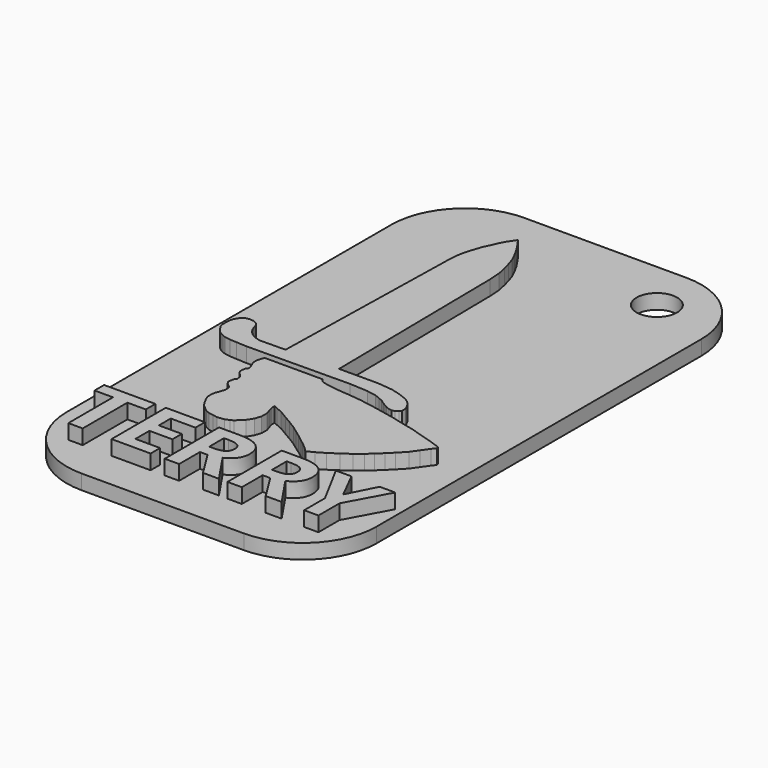
from build123d import *

# Parameters (mm, degrees)
F1_DEPTH     = 2
F3_DEPTH     = 2
F4_TEXT_SIZE = 12.8735775231
F5_DEPTH     = 2
F6_R         = 2.75
F7_DEPTH     = 25


# Not quite as in the source:
# - Text() gives the source's letters only with a copy of the font that has no kerning and outlines rounded to 1/6400 em; it was checked with that copy


with BuildPart() as f1:
    # F0 (on Top) → F1 (new body)
    with BuildSketch(Plane.XY):
        with BuildLine():
            Line((-32, 0), (-10, 0))
            ThreePointArc((-10, 0), (-2.9289321881, 2.9289321881), (0, 10))
            Line((0, 10), (0, 65))
            ThreePointArc((0, 65), (-2.9289321881, 72.0710678119), (-10, 75))
            Line((-10, 75), (-32, 75))
            ThreePointArc((-32, 75), (-39.0710678119, 72.0710678119), (-42, 65))
            Line((-42, 65), (-42, 10))
            ThreePointArc((-42, 10), (-39.0710678119, 2.9289321881), (-32, 0))
        make_face()
    extrude(amount=F1_DEPTH)

    # F2 (on face) → F3 (join)
    with BuildSketch(Plane.XY.offset(2)):
        Polygon((-24.9658841423, 16.3784821588), (-24.6103350073, 16.5639445186), (-23.6864611506, 17.4445118755), (-23.1667812914, 18.2529017329), (-22.8780712932, 19.11903359), (-22.8780712932, 20.0573448092), (-23.1523457915, 20.8657346666), (-23.2822652906, 21.4142855257), (-23.2822652906, 21.8184795231), (-22.8058937937, 21.6019470245), (-21.8964535743, 21.212188527), (-20.8426602185, 20.5770246685), (-19.7022520006, 19.9129898101), (-18.7206342816, 19.3066969514), (-17.8978089243, 18.7004040927), (-17.0172415674, 18.079675734), (-16.2377227098, 17.4589473754), (-15.6025588512, 16.9825740159), (-14.7941680625, 16.3041036576), (-14.2744891346, 15.7555527985), (-13.3170420304, 16.2503849715), (-12.2686894611, 16.8681629002), (-11.0705727711, 17.6731478423), (-9.9660586566, 18.4406917542), (-9.0113086626, 19.2082356662), (-8.2063237205, 19.9383385479), (-7.4123837985, 20.6902306527), (-6.6134268418, 21.4891862124), (-5.6124022231, 22.5375965238), (-4.9415803514, 23.4873015434), (-4.2178332806, 24.5201177895), (-3.8306072117, 25.0064013927), (-3.9369123988, 25.3037977964), (-5.5035836995, 25.836231187), (-6.8984818645, 26.2547004968), (-8.5956072435, 26.7777871341), (-10.4554714635, 27.219504118), (-11.9201140478, 27.5914780796), (-13.6976763606, 27.9617961496), (-15.6040368602, 28.3337701112), (-17.184920609, 28.5895001143), (-18.7076851726, 28.752239421), (-20.2072001994, 28.8801044226), (-21.7415876687, 29.0777143091), (-22.498941049, 29.2605310678), (-22.8733532131, 29.4102951884), (-23.1916029006, 29.7847073525), (-31.0095064342, 29.7847073525), (-31.1390943825, 29.3874349445), (-31.2969014049, 28.8715362549), (-31.2969014049, 28.5498574376), (-31.2969014049, 28.1856935471), (-31.1026796699, 27.7608353645), (-30.9327356517, 27.3602548987), (-30.8599025011, 27.1538961679), (-30.8599025011, 26.8261488527), (-31.0598810524, 26.575013151), (-31.130105257, 26.1785797775), (-31.130105257, 25.8173905313), (-31.0041401535, 25.5104210228), (-30.7050403208, 25.2034496516), (-30.4604899138, 24.9401368201), (-30.3138699383, 24.7593056411), (-30.3138699383, 24.5201177895), (-30.2734393626, 24.2165140808), (-30.4760091814, 23.9621242313), (-30.5441141428, 23.5776545209), (-30.6210232253, 23.1434833228), (-30.4369907826, 22.8033997118), (-30.1447939128, 22.5287377834), (-29.8052169383, 22.2937427461), (-29.6849943697, 21.9772327691), (-29.6849943697, 21.4689467102), (-29.8709366471, 20.8725202829), (-30.0894360989, 20.3019957989), (-30.184677618, 19.7643333657), (-30.184677618, 19.1148594022), (-29.9427583814, 18.5079202056), (-29.5939017087, 17.877869308), (-29.2224623263, 17.2620639205), (-28.7184887627, 16.8607513931), (-28.2475364605, 16.4857335899), (-27.7093555778, 16.2511784583), (-27.085136602, 16.140604314), (-26.4370755417, 16.025806783), (-25.5564892781, 16.1430734978), align=None)
        Polygon((-23.2822652906, 32.7390320599), (-23.2822652906, 32.8520275652), (-23.6235633492, 58.7551258504), (-23.7346049398, 60.4145303369), (-24.0059494972, 61.6808012128), (-24.2672394961, 62.634550035), (-24.6103350073, 63.719920814), (-25.0998698175, 64.7255629301), (-25.6353718438, 65.6927037613), (-26.137124747, 66.4726048708), (-26.9337110221, 67.622564733), (-27.622455731, 66.6155517101), (-28.0409250408, 65.8483579755), (-28.4128971398, 65), (-28.9243590087, 63.9071241021), (-29.2009095763, 63.0200635078), (-29.3751433492, 62.5206828117), (-29.4680605514, 62.2226426039), (-29.6321341877, 61.5429361925), (-29.7384271195, 60.9428857426), (-29.8511039958, 59.621486868), (-30.4369907826, 32.8768156469), (-30.4369907826, 32.6301716268), (-33.9809825375, 32.5834761508), (-34.709648225, 32.8106454228), (-35.3001132607, 33.1588685513), (-35.7344733009, 33.5671623373), (-36.0429808497, 34.0070165694), (-36.2483075647, 34.5221505998), (-36.4160070111, 35.0526619962), (-36.7120355689, 35.4177636334), (-37.1375491344, 35.6687076454), (-37.7274300119, 35.7190073209), (-38.2593304964, 35.6481747121), (-38.6143550277, 35.4177636334), (-38.9050842869, 35.0526619962), (-39.1125643774, 34.7008480899), (-39.2378741141, 34.2989059409), (-39.2978957527, 33.7372787216), (-39.2884454103, 33.0200371736), (-39.2004437745, 32.6014347374), (-38.9972887933, 32.2722643614), (-38.7773551047, 31.9350361824), (-38.4736694396, 31.5763056278), (-38.1266660988, 31.2928371131), (-37.6965813339, 31.0631338507), (-37.2469425201, 30.8871883899), (-36.5124084055, 30.775571242), (-35.5935879052, 30.7266972959), (-34.1448035996, 30.6496334886), (-20.2175881714, 30.7756159455), (-17.7779836218, 30.6458483781), (-16.442425549, 30.4053537548), (-15.837890952, 30.1687969563), (-15.2122387663, 29.8731327057), (-14.7084929049, 29.5228715986), (-14.3009340391, 29.2632207274), (-13.8530861831, 29.024030405), (-13.4119355894, 28.8514064186), (-12.9810938237, 28.7859372618), (-12.6245720312, 28.9015565068), (-12.2919679692, 29.1184744358), (-12.0967384428, 29.3854027987), (-12.0673207199, 29.9384501587), (-12.2384717688, 30.3677618504), (-12.5316884369, 30.8892671019), (-12.9265692085, 31.3324257731), (-13.3319823063, 31.6289420603), (-13.8487648219, 31.8711660802), (-14.5679111264, 32.1525708969), (-15.2193773538, 32.3426537216), (-15.9513838589, 32.5394310057), (-16.8093256652, 32.6181389391), (-17.9284624755, 32.7390320599), align=None)
    extrude(amount=F3_DEPTH)

    # F4 (on face) → F5 (join)
    with BuildSketch(Plane.XY.offset(2)):
        with Locations((-40.6403224915, 5.1358705387)):
            Text('TERRY', F4_TEXT_SIZE, font='Open Sans', font_style=FontStyle.BOLD, text_align=(TextAlign.LEFT, TextAlign.BOTTOM))
    extrude(amount=F5_DEPTH)

    # F6 (on face) → F7 (cut)
    with BuildSketch(Plane.XY.offset(2)):
        with Locations((-8.5590155795, 68.1730508804)):
            Circle(F6_R)
    extrude(amount=-F7_DEPTH, mode=Mode.SUBTRACT)


solid = f1.part
